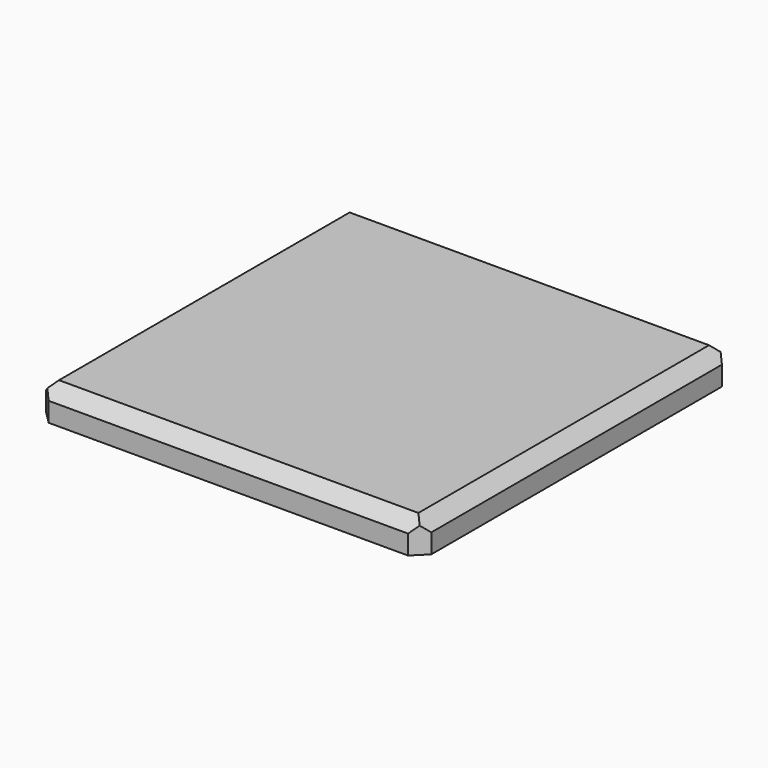
from build123d import *

# Parameters (mm, degrees)
F0_W     = 151.572406292
F0_H     = 153.1009078026
F1_DEPTH = 6.35
F2_SIZE  = 5.08
F3_SIZE  = 5.08
F4_SIZE  = 5.08
F5_SIZE  = 5.08
F6_W     = 17.9464835674
F6_H     = 13.5393217206
F7_DEPTH = 0.762
F8_W     = 21.0372619331
F8_H     = 13.5393217206
F9_DEPTH = 0.762
F10_SIZE = 5.08
F11_SIZE = 5.08
F12_SIZE = 5.08
F13_SIZE = 5.08


with BuildPart() as f1:
    # F0 (on Top) → F1 (new body, symmetric)
    with BuildSketch(Plane.XY):
        with Locations((-0.1000165939, 0.1238584518)):
            Rectangle(F0_W, F0_H)
    extrude(amount=F1_DEPTH, both=True)

    # F2
    f2_edges = [f1.edges().sort_by_distance(p)[0] for p in [
        (-0.100017, -76.426595, 6.35),
    ]]
    chamfer(f2_edges, length=F2_SIZE)

    # F3
    f3_edges = [f1.edges().sort_by_distance(p)[0] for p in [
        (-0.100017, 76.674312, 6.35),
    ]]
    chamfer(f3_edges, length=F3_SIZE)

    # F4
    f4_edges = [f1.edges().sort_by_distance(p)[0] for p in [
        (75.686187, 0.123858, 6.35),
    ]]
    chamfer(f4_edges, length=F4_SIZE)

    # F5
    f5_edges = [f1.edges().sort_by_distance(p)[0] for p in [
        (-75.88622, 0.123858, 6.35),
    ]]
    chamfer(f5_edges, length=F5_SIZE)

    # F6 (on face) → F7 (cut)
    with BuildSketch(Plane(origin=(0, 0, -6.35), x_dir=(1, 0, 0), z_dir=(0, 0, -1))):
        with Locations((32.9451402649, -69.9046514928)):
            Rectangle(F6_W, F6_H)
    extrude(amount=-F7_DEPTH, mode=Mode.SUBTRACT)

    # F8 (on face) → F9 (cut)
    with BuildSketch(Plane(origin=(0, 0, -6.35), x_dir=(1, 0, 0), z_dir=(0, 0, -1))):
        with Locations((-35.0907575339, -69.9046514928)):
            Rectangle(F8_W, F8_H)
    extrude(amount=-F9_DEPTH, mode=Mode.SUBTRACT)

    # F10
    f10_edges = [f1.edges().sort_by_distance(p)[0] for p in [
        (75.686187, -76.426595, -2.54),
    ]]
    chamfer(f10_edges, length=F10_SIZE)

    # F11
    f11_edges = [f1.edges().sort_by_distance(p)[0] for p in [
        (75.686187, 76.674312, -2.54),
    ]]
    chamfer(f11_edges, length=F11_SIZE)

    # F12
    f12_edges = [f1.edges().sort_by_distance(p)[0] for p in [
        (-75.88622, 76.674312, -2.54),
    ]]
    chamfer(f12_edges, length=F12_SIZE)

    # F13
    f13_edges = [f1.edges().sort_by_distance(p)[0] for p in [
        (-75.88622, -76.426595, -2.54),
    ]]
    chamfer(f13_edges, length=F13_SIZE)


solid = f1.part
